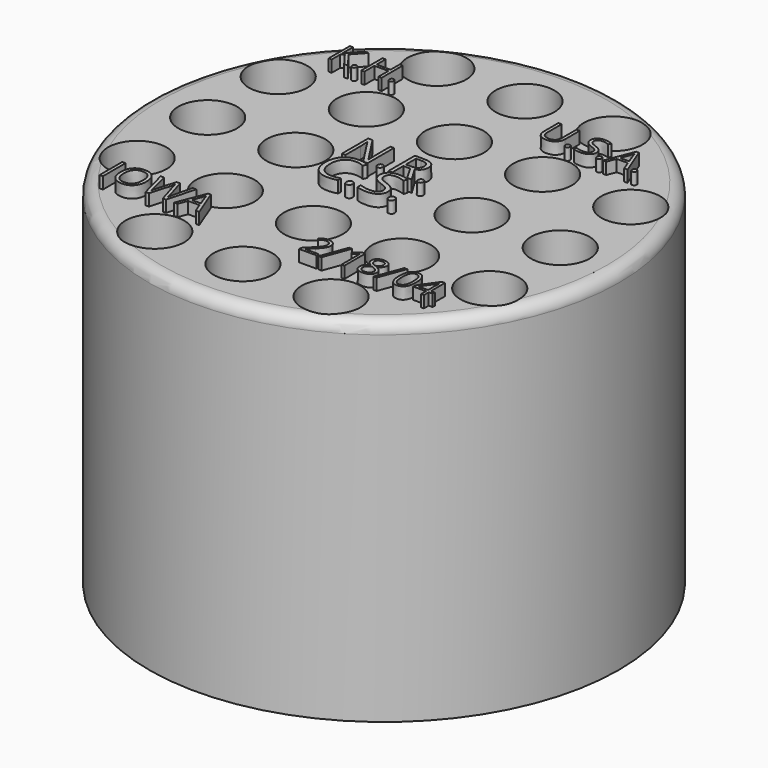
from build123d import *

# Parameters (mm, degrees)
F0_R           = 50.8
F1_DEPTH       = 50.8
F1_DEPTH_BACK  = 25.4
F2_R           = 6.35
F3_DEPTH       = 50.8
F4_TEXT_SIZE   = 9.9890915374
F4_TEXT_SIZE_2 = 11.3046070061
F4_TEXT_SIZE_3 = 11.2973321747
F5_DEPTH       = 2.54
F6_TEXT_SIZE   = 8.031909561
F7_DEPTH       = 2.54
F8_TEXT_SIZE   = 8.4008116068
F9_DEPTH       = 2.54
F10_TEXT_SIZE  = 8.5533389615
F11_DEPTH      = 2.54
F12_TEXT_SIZE  = 7.8932330426
F13_DEPTH      = 2.54


# Not quite as in the source:
# - a fillet or chamfer that OpenCascade refuses, or shapes differently, is made with other operations: its cross-section is extruded or revolved along the edge and cut away or added
# - a feature names something its author has since deleted; it is built from what else it names
# - Text() gives the source's letters only with a copy of the font that has no kerning and outlines rounded to 1/6400 em; it was checked with that copy


with BuildPart() as f1:
    # F0 (on Top) → F1 (new body, two sides)
    with BuildSketch(Plane.XY) as f1_sk:
        Circle(F0_R)
    extrude(amount=F1_DEPTH)
    extrude(f1_sk.sketch, amount=-F1_DEPTH_BACK)

    # F2 (on face) → F3 (cut)
    with BuildSketch(Plane.XY.offset(50.8)):
        with Locations((38.1, 19.05)):
            Circle(F2_R)
        with Locations((19.05, 38.1)):
            Circle(F2_R)
        with Locations((19.05, 19.05)):
            Circle(F2_R)
        with Locations((19.05, 0)):
            Circle(F2_R)
        with Locations((0, 19.05)):
            Circle(F2_R)
        with Locations((0, 38.1)):
            Circle(F2_R)
        with Locations((-19.05, 38.1)):
            Circle(F2_R)
        with Locations((-19.05, 19.05)):
            Circle(F2_R)
        with Locations((-38.1, 19.05)):
            Circle(F2_R)
        with Locations((-38.1, 0)):
            Circle(F2_R)
        with Locations((-19.05, 0)):
            Circle(F2_R)
        with Locations((0, -19.05)):
            Circle(F2_R)
        with Locations((-19.05, -19.05)):
            Circle(F2_R)
        with Locations((-38.1, -19.05)):
            Circle(F2_R)
        with Locations((19.05, -19.05)):
            Circle(F2_R)
        with Locations((19.05, -38.1)):
            Circle(F2_R)
        with Locations((0, -38.1)):
            Circle(F2_R)
        with Locations((-19.05, -38.1)):
            Circle(F2_R)
        with Locations((38.1, -19.05)):
            Circle(F2_R)
        with Locations((38.1, 0)):
            Circle(F2_R)
    extrude(amount=-F3_DEPTH, mode=Mode.SUBTRACT)

    # F4 (on face) → F5 (join)
    with BuildSketch(Plane.XY.offset(50.8)):
        with Locations((-10.095225635, 0)):
            Text('N.', F4_TEXT_SIZE, font='Open Sans', text_align=(TextAlign.LEFT, TextAlign.BOTTOM))
        with Locations((0, 0)):
            Text('R.', F4_TEXT_SIZE, font='Open Sans', text_align=(TextAlign.LEFT, TextAlign.BOTTOM))
        with Locations((-10.0346050628, -8.1393170444)):
            Text('C.', F4_TEXT_SIZE_2, font='Open Sans', text_align=(TextAlign.LEFT, TextAlign.BOTTOM))
        with Locations((0, -8.1340791658)):
            Text('S.', F4_TEXT_SIZE_3, font='Open Sans', text_align=(TextAlign.LEFT, TextAlign.BOTTOM))
    extrude(amount=F5_DEPTH)

    # F6 (on face) → F7 (join)
    with BuildSketch(Plane.XY.offset(50.8)):
        with Locations((-33.4065146744, 25.8270483464)):
            Text('K.H.', F6_TEXT_SIZE, font='Open Sans', text_align=(TextAlign.LEFT, TextAlign.BOTTOM))
    extrude(amount=F7_DEPTH)

    # F8 (on face) → F9 (join)
    with BuildSketch(Plane.XY.offset(50.8)):
        with Locations((11.6662411019, 25.5864690989)):
            Text('U.S.A.', F8_TEXT_SIZE, font='Open Sans', text_align=(TextAlign.LEFT, TextAlign.BOTTOM))
    extrude(amount=F9_DEPTH)

    # F10 (on face) → F11 (join)
    with BuildSketch(Plane.XY.offset(50.8)):
        with Locations((-37.0021760464, -31.6272899508)):
            Text('IOWA', F10_TEXT_SIZE, font='Open Sans', text_align=(TextAlign.LEFT, TextAlign.BOTTOM))
    extrude(amount=F11_DEPTH)

    # F12 (on face) → F13 (join)
    with BuildSketch(Plane.XY.offset(50.8)):
        with Locations((6.6332035931, -31.6970366985)):
            Text('2/18/04', F12_TEXT_SIZE, font='Open Sans', text_align=(TextAlign.LEFT, TextAlign.BOTTOM))
    extrude(amount=F13_DEPTH)

    # F14: fillet of radius 2.54 on 1 edges, made by hand

    # F14_s1 → F14_t2 (revolve, cut)
    with BuildSketch(Plane.XZ):
        with BuildLine():
            ThreePointArc((50.8, 48.26), (50.0560512242, 50.0560512242), (48.26, 50.8))
            Line((48.26, 50.8), (50.8, 50.8))
            Line((50.8, 50.8), (50.8, 48.26))
        make_face()
    revolve(axis=Axis((0, 0, 50.8), (0, 0, 1)), mode=Mode.SUBTRACT)


solid = f1.part
